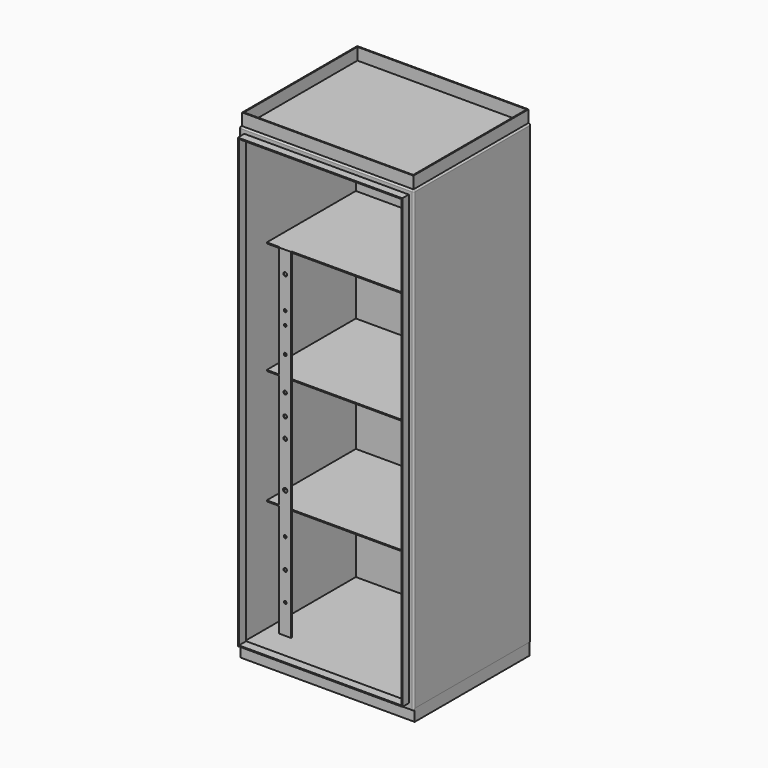
from build123d import *

# Parameters (mm, degrees)
F0_W          = 546.1
F0_H          = 1438.275
F1_DEPTH      = 3.175
F3_W          = 457.2
F3_H          = 1438.275
F4_DEPTH      = 3.175
F6_W          = 457.2
F6_H          = 1438.275
F7_DEPTH      = 3.175
F8_W          = 552.45
F8_H          = 457.2
F9_DEPTH      = 3.175
F10_W         = 546.1
F10_H         = 352.4375557899
F11_DEPTH     = 1.5875
F12_W         = 546.1
F12_H         = 352.425
F13_DEPTH     = 1.5875
F15_W         = 546.1
F15_H         = 352.425
F16_DEPTH     = 1.5875
F17_W         = 552.45
F17_H         = 457.2
F18_DEPTH     = 3.175
F20_DEPTH     = 2.54
F21_W         = 552.45
F21_H         = 1449.705
F21_W_2       = 514.35
F21_H_2       = 1411.605
F22_DEPTH     = 3.175
F23_W         = 520.7
F23_H         = 1417.955
F23_W_2       = 514.35
F23_H_2       = 1411.605
F24_DEPTH     = 25.4
F25_R         = 5.08
F26_T1_DEPTH  = 467.995
F26_S5_W      = 5.08
F26_S5_H      = 5.08
F26_T6_DEPTH  = 5.08
F26_S11_W     = 5.08
F26_S11_H     = 5.08
F26_T12_DEPTH = 5.08
F27_W         = 551.4826476574
F27_H         = 455.4039281793
F27_W_2       = 545.4865694046
F27_H_2       = 449.852083344
F28_DEPTH     = 38.1
F29_DEPTH     = 38.1
F30_W         = 542.29
F30_H         = 455.295
F30_W_2       = 535.94
F30_H_2       = 448.945
F31_DEPTH     = 38.1


# Not quite as in the source:
# - a fillet or chamfer that OpenCascade refuses, or shapes differently, is made with other operations: its cross-section is extruded or revolved along the edge and cut away or added


with BuildPart() as f1:
    # F0 (on Front) → F1 (new body)
    with BuildSketch(Plane.XZ):
        Rectangle(F0_W, F0_H)
    extrude(amount=-F1_DEPTH)

    # F3 (on face) → F4 (join)
    with BuildSketch(Plane.YZ.offset(273.05)):
        with Locations((-225.425, 0)):
            Rectangle(F3_W, F3_H)
    extrude(amount=F4_DEPTH)

    # F6 (on face) → F7 (join)
    with BuildSketch(Plane(origin=(-273.05, 0, 0), x_dir=(0, -1, 0), z_dir=(-1, 0, 0))):
        with Locations((225.425, 0)):
            Rectangle(F6_W, F6_H)
    extrude(amount=F7_DEPTH)

    # F8 (on face) → F9 (join)
    with BuildSketch(Plane(origin=(0, 0, -719.1375), x_dir=(1, 0, 0), z_dir=(0, 0, -1))):
        with Locations((0, 225.425)):
            Rectangle(F8_W, F8_H)
    extrude(amount=F9_DEPTH)

    # F10 (on offset) → F11 (join, symmetric)
    with BuildSketch(Plane.XY.offset(-363.5375)):
        with Locations((0, -176.218777895)):
            Rectangle(F10_W, F10_H)
    extrude(amount=F11_DEPTH, both=True)

    # F12 (on Top) → F13 (join, symmetric)
    with BuildSketch(Plane.XY):
        with Locations((0, -176.2125)):
            Rectangle(F12_W, F12_H)
    extrude(amount=F13_DEPTH, both=True)

    # F15 (on offset) → F16 (join, symmetric)
    with BuildSketch(Plane.XY.offset(355.6)):
        with Locations((0, -176.2125)):
            Rectangle(F15_W, F15_H)
    extrude(amount=F16_DEPTH, both=True)

    # F17 (on face) → F18 (join)
    with BuildSketch(Plane.XY.offset(719.1375)):
        with Locations((0, -225.425)):
            Rectangle(F17_W, F17_H)
    extrude(amount=F18_DEPTH)

    # F19 (on face) → F20 (join)
    with BuildSketch(Plane.XZ.offset(352.425)):
        with BuildLine():
            Line((-212.725, 357.1875), (-231.775, 357.1875))
            Line((-231.775, 357.1875), (-231.775, -719.3357628388))
            Line((-231.775, -719.3357628388), (-212.725, -719.3357628388))
            Line((-212.725, -719.3357628388), (-212.725, -630.4557702019))
            ThreePointArc((-212.725, -630.4557702019), (-217.117602153, -626.0631680489), (-212.725, -621.6705658958))
            Line((-212.725, -621.6705658958), (-212.725, -540.6397135398))
            ThreePointArc((-212.725, -540.6397135398), (-218.1377724311, -535.2269411087), (-212.725, -529.8141686776))
            Line((-212.725, -529.8141686776), (-212.725, -447.3259880815))
            ThreePointArc((-212.725, -447.3259880815), (-217.2657846247, -442.7852034569), (-212.725, -438.2444188322))
            Line((-212.725, -438.2444188322), (-212.725, -320.1060615697))
            ThreePointArc((-212.725, -320.1060615697), (-219.4191999116, -313.4118616581), (-212.725, -306.7176617465))
            Line((-212.725, -306.7176617465), (-212.725, -175.5880119798))
            ThreePointArc((-212.725, -175.5880119798), (-218.4829877374, -169.8300242424), (-212.725, -164.072036505))
            Line((-212.725, -164.072036505), (-212.725, -113.2661164384))
            ThreePointArc((-212.725, -113.2661164384), (-218.4185534458, -107.5725629926), (-212.725, -101.8790095467))
            Line((-212.725, -101.8790095467), (-212.725, -46.6509112122))
            ThreePointArc((-212.725, -46.6509112122), (-218.1210778716, -41.2548333406), (-212.725, -35.8587554691))
            Line((-212.725, -35.8587554691), (-212.725, 60.6955810605))
            ThreePointArc((-212.725, 60.6955810605), (-217.3495903553, 65.3201714158), (-212.725, 69.9447617711))
            Line((-212.725, 69.9447617711), (-212.725, 142.4734210846))
            ThreePointArc((-212.725, 142.4734210846), (-216.7484708908, 146.4968919754), (-212.725, 150.5203628662))
            Line((-212.725, 150.5203628662), (-212.725, 183.0033609852))
            ThreePointArc((-212.725, 183.0033609852), (-217.0262847916, 187.3046457767), (-212.725, 191.6059305683))
            Line((-212.725, 191.6059305683), (-212.725, 283.1353669526))
            ThreePointArc((-212.725, 283.1353669526), (-218.6943033336, 289.1046702862), (-212.725, 295.0739736198))
            Line((-212.725, 295.0739736198), (-212.725, 357.1875))
        make_face()
        with BuildLine():
            Line((-193.675, 357.1875), (-212.725, 357.1875))
            Line((-212.725, 357.1875), (-212.725, 295.0739736198))
            ThreePointArc((-212.725, 295.0739736198), (-208.5040651339, 293.3256051523), (-206.7556966664, 289.1046702862))
            ThreePointArc((-206.7556966664, 289.1046702862), (-208.5040651339, 284.88373542), (-212.725, 283.1353669526))
            Line((-212.725, 283.1353669526), (-212.725, 191.6059305683))
            ThreePointArc((-212.725, 191.6059305683), (-209.6835323561, 190.3461134207), (-208.4237152084, 187.3046457767))
            ThreePointArc((-208.4237152084, 187.3046457767), (-209.6835323561, 184.2631781328), (-212.725, 183.0033609852))
            Line((-212.725, 183.0033609852), (-212.725, 150.5203628662))
            ThreePointArc((-212.725, 150.5203628662), (-209.8799764492, 149.3419155262), (-208.7015291092, 146.4968919754))
            ThreePointArc((-208.7015291092, 146.4968919754), (-209.8799764492, 143.6518684246), (-212.725, 142.4734210846))
            Line((-212.725, 142.4734210846), (-212.725, 69.9447617711))
            ThreePointArc((-212.725, 69.9447617711), (-209.4549207996, 68.5902506162), (-208.1004096447, 65.3201714158))
            ThreePointArc((-208.1004096447, 65.3201714158), (-209.4549207996, 62.0500922154), (-212.725, 60.6955810605))
            Line((-212.725, 60.6955810605), (-212.725, -35.8587554691))
            ThreePointArc((-212.725, -35.8587554691), (-208.9093967452, -37.4392300858), (-207.3289221284, -41.2548333406))
            ThreePointArc((-207.3289221284, -41.2548333406), (-208.9093967452, -45.0704365955), (-212.725, -46.6509112122))
            Line((-212.725, -46.6509112122), (-212.725, -101.8790095467))
            ThreePointArc((-212.725, -101.8790095467), (-208.6990497494, -103.546612742), (-207.0314465542, -107.5725629926))
            ThreePointArc((-207.0314465542, -107.5725629926), (-208.6990497494, -111.5985132432), (-212.725, -113.2661164384))
            Line((-212.725, -113.2661164384), (-212.725, -164.072036505))
            ThreePointArc((-212.725, -164.072036505), (-208.6534878249, -165.7585120673), (-206.9670122626, -169.8300242424))
            ThreePointArc((-206.9670122626, -169.8300242424), (-208.6534878249, -173.9015364175), (-212.725, -175.5880119798))
            Line((-212.725, -175.5880119798), (-212.725, -306.7176617465))
            ThreePointArc((-212.725, -306.7176617465), (-207.9914858479, -308.678347506), (-206.0308000884, -313.4118616581))
            ThreePointArc((-206.0308000884, -313.4118616581), (-207.9914858479, -318.1453758102), (-212.725, -320.1060615697))
            Line((-212.725, -320.1060615697), (-212.725, -438.2444188322))
            ThreePointArc((-212.725, -438.2444188322), (-209.5141804, -439.5743838569), (-208.1842153753, -442.7852034569))
            ThreePointArc((-208.1842153753, -442.7852034569), (-209.5141804, -445.9960230569), (-212.725, -447.3259880815))
            Line((-212.725, -447.3259880815), (-212.725, -529.8141686776))
            ThreePointArc((-212.725, -529.8141686776), (-208.8975919089, -531.3995330176), (-207.3122275689, -535.2269411087))
            ThreePointArc((-207.3122275689, -535.2269411087), (-208.8975919089, -539.0543491998), (-212.725, -540.6397135398))
            Line((-212.725, -540.6397135398), (-212.725, -621.6705658958))
            ThreePointArc((-212.725, -621.6705658958), (-209.6189612305, -622.9571292794), (-208.332397847, -626.0631680489))
            ThreePointArc((-208.332397847, -626.0631680489), (-209.6189612305, -629.1692068183), (-212.725, -630.4557702019))
            Line((-212.725, -630.4557702019), (-212.725, -719.3357628388))
            Line((-212.725, -719.3357628388), (-193.675, -719.3357628388))
            Line((-193.675, -719.3357628388), (-193.675, 357.1875))
        make_face()
        with BuildLine():
            Line((231.775, -719.3357628388), (231.775, 357.1875))
            Line((231.775, 357.1875), (212.725, 357.1875))
            Line((212.725, 357.1875), (212.725, 295.2589705741))
            ThreePointArc((212.725, 295.2589705741), (217.0767474671, 293.4564177533), (218.879300288, 289.1046702862))
            ThreePointArc((218.879300288, 289.1046702862), (217.0767474671, 284.7529228191), (212.725, 282.9503699982))
            Line((212.725, 282.9503699982), (212.725, 195.2587648768))
            ThreePointArc((212.725, 195.2587648768), (218.349411554, 192.9290573307), (220.6791191, 187.3046457767))
            ThreePointArc((220.6791191, 187.3046457767), (218.349411554, 181.6802342227), (212.725, 179.3505266767))
            Line((212.725, 179.3505266767), (212.725, 152.5461312326))
            ThreePointArc((212.725, 152.5461312326), (217.0024580998, 150.7743500752), (218.7742392572, 146.4968919754))
            ThreePointArc((218.7742392572, 146.4968919754), (217.0024580998, 142.2194338756), (212.725, 140.4476527182))
            Line((212.725, 140.4476527182), (212.725, 72.6305128958))
            ThreePointArc((212.725, 72.6305128958), (217.8941920333, 70.4893634491), (220.03534148, 65.3201714158))
            ThreePointArc((220.03534148, 65.3201714158), (217.8941920333, 60.1509793825), (212.725, 58.0098299358))
            Line((212.725, 58.0098299358), (212.725, -35.4249250966))
            ThreePointArc((212.725, -35.4249250966), (216.847367653, -37.1324656876), (218.554908244, -41.2548333406))
            ThreePointArc((218.554908244, -41.2548333406), (216.847367653, -45.3772009937), (212.725, -47.0847415846))
            Line((212.725, -47.0847415846), (212.725, -102.0553301101))
            ThreePointArc((212.725, -102.0553301101), (216.6262727846, -103.671290208), (218.2422328825, -107.5725629926))
            ThreePointArc((218.2422328825, -107.5725629926), (216.6262727846, -111.4738357772), (212.725, -113.089795875))
            Line((212.725, -113.089795875), (212.725, -162.3801945495))
            ThreePointArc((212.725, -162.3801945495), (217.9928250946, -164.5621991478), (220.1748296929, -169.8300242424))
            ThreePointArc((220.1748296929, -169.8300242424), (217.9928250946, -175.097849337), (212.725, -177.2798539353))
            Line((212.725, -177.2798539353), (212.725, -306.509428103))
            ThreePointArc((212.725, -306.509428103), (217.6057575735, -308.5311040846), (219.6274335551, -313.4118616581))
            ThreePointArc((219.6274335551, -313.4118616581), (217.6057575735, -318.2926192316), (212.725, -320.3142952132))
            Line((212.725, -320.3142952132), (212.725, -436.1559807838))
            ThreePointArc((212.725, -436.1559807838), (217.4125683061, -438.0976351507), (219.3542226731, -442.7852034569))
            ThreePointArc((219.3542226731, -442.7852034569), (217.4125683061, -447.472771763), (212.725, -449.41442613))
            Line((212.725, -449.41442613), (212.725, -528.9798604641))
            ThreePointArc((212.725, -528.9798604641), (217.1423530864, -530.8095880223), (218.9720806446, -535.2269411087))
            ThreePointArc((218.9720806446, -535.2269411087), (217.1423530864, -539.6442941951), (212.725, -541.4740217533))
            Line((212.725, -541.4740217533), (212.725, -619.9717660694))
            ThreePointArc((212.725, -619.9717660694), (217.0322716466, -621.7558964023), (218.8164019794, -626.0631680489))
            ThreePointArc((218.8164019794, -626.0631680489), (217.0322716466, -630.3704396954), (212.725, -632.1545700283))
            Line((212.725, -632.1545700283), (212.725, -719.3357628388))
            Line((212.725, -719.3357628388), (231.775, -719.3357628388))
        make_face()
        with BuildLine():
            Line((212.725, 295.2589705741), (212.725, 357.1875))
            Line((212.725, 357.1875), (193.675, 357.1875))
            Line((193.675, 357.1875), (193.675, -719.3357628388))
            Line((193.675, -719.3357628388), (212.725, -719.3357628388))
            Line((212.725, -719.3357628388), (212.725, -632.1545700283))
            ThreePointArc((212.725, -632.1545700283), (206.6335980206, -626.0631680489), (212.725, -619.9717660694))
            Line((212.725, -619.9717660694), (212.725, -541.4740217533))
            ThreePointArc((212.725, -541.4740217533), (206.4779193554, -535.2269411087), (212.725, -528.9798604641))
            Line((212.725, -528.9798604641), (212.725, -449.41442613))
            ThreePointArc((212.725, -449.41442613), (206.0957773269, -442.7852034569), (212.725, -436.1559807838))
            Line((212.725, -436.1559807838), (212.725, -320.3142952132))
            ThreePointArc((212.725, -320.3142952132), (205.8225664449, -313.4118616581), (212.725, -306.509428103))
            Line((212.725, -306.509428103), (212.725, -177.2798539353))
            ThreePointArc((212.725, -177.2798539353), (205.2751703071, -169.8300242424), (212.725, -162.3801945495))
            Line((212.725, -162.3801945495), (212.725, -113.089795875))
            ThreePointArc((212.725, -113.089795875), (207.2077671175, -107.5725629926), (212.725, -102.0553301101))
            Line((212.725, -102.0553301101), (212.725, -47.0847415846))
            ThreePointArc((212.725, -47.0847415846), (206.895091756, -41.2548333406), (212.725, -35.4249250966))
            Line((212.725, -35.4249250966), (212.725, 58.0098299358))
            ThreePointArc((212.725, 58.0098299358), (205.41465852, 65.3201714158), (212.725, 72.6305128958))
            Line((212.725, 72.6305128958), (212.725, 140.4476527182))
            ThreePointArc((212.725, 140.4476527182), (206.6757607428, 146.4968919754), (212.725, 152.5461312326))
            Line((212.725, 152.5461312326), (212.725, 179.3505266767))
            ThreePointArc((212.725, 179.3505266767), (204.7708809, 187.3046457767), (212.725, 195.2587648768))
            Line((212.725, 195.2587648768), (212.725, 282.9503699982))
            ThreePointArc((212.725, 282.9503699982), (206.570699712, 289.1046702862), (212.725, 295.2589705741))
        make_face()
    extrude(amount=F20_DEPTH)

    # F21 (on face) → F22 (join)
    with BuildSketch(Plane.XZ.offset(454.025)):
        with Locations((0, -2.54)):
            Rectangle(F21_W, F21_H)
        with Locations((0, -2.54)):
            Rectangle(F21_W_2, F21_H_2, mode=Mode.SUBTRACT)
    extrude(amount=F22_DEPTH)

    # F23 (on face) → F24 (join)
    with BuildSketch(Plane.XZ.offset(457.2)):
        with Locations((0, -2.54)):
            Rectangle(F23_W, F23_H)
        with Locations((0, -2.54)):
            Rectangle(F23_W_2, F23_H_2, mode=Mode.SUBTRACT)
    extrude(amount=F24_DEPTH)

    # F25
    f25_edges = [f1.edges().sort_by_distance(p)[0] for p in [
        (0, -457.2, 722.3125),
        (276.225, -457.2, -2.54),
        (-276.225, -457.2, -2.54),
    ]]
    fillet(f25_edges, radius=F25_R)

    # F26: fillet of radius 5.08 on 2 edges, made by hand

    # F26_s2 → F26_t1 (cut)
    with BuildSketch(Plane.XZ.offset(-15.875)):
        with BuildLine():
            ThreePointArc((276.225, 717.2325), (274.7371024484, 720.8246024484), (271.145, 722.3125))
            Line((271.145, 722.3125), (276.225, 722.3125))
            Line((276.225, 722.3125), (276.225, 717.2325))
        make_face()
        with BuildLine():
            ThreePointArc((-276.225, 717.2325), (-274.7371024484, 720.8246024484), (-271.145, 722.3125))
            Line((-271.145, 722.3125), (-276.225, 722.3125))
            Line((-276.225, 722.3125), (-276.225, 717.2325))
        make_face()
    extrude(amount=F26_T1_DEPTH, mode=Mode.SUBTRACT)


with BuildPart() as f26_tool4:
    # F26_s5 → F26_t6 (new body)
    with BuildSketch(Plane.YZ.offset(-271.145)):
        with Locations((-454.66, 719.7725)):
            Rectangle(F26_S5_W, F26_S5_H)
    extrude(amount=-F26_T6_DEPTH)

    # F26_s7 → F26_t8 (revolve, cut)
    with BuildSketch(Plane(origin=(-271.145, -452.12, 717.2325), x_dir=(0, 0.7071067812, -0.7071067812), z_dir=(0, 0.7071067812, 0.7071067812))):
        with BuildLine():
            ThreePointArc((0, -5.08), (5.08, 0), (0, 5.08))
            Line((0, 5.08), (0, -5.08))
        make_face()
    revolve(axis=Axis((-271.145, -452.12, 717.2325), (-1, 0, 0)), mode=Mode.SUBTRACT)


with BuildPart() as f1_1:
    add(f1.part)

    # F26_t3: cut F26_tool4
    add(f26_tool4.part, mode=Mode.SUBTRACT)


with BuildPart() as f26_tool10:
    # F26_s11 → F26_t12 (new body)
    with BuildSketch(Plane.YZ.offset(271.145)):
        with Locations((-454.66, 719.7725)):
            Rectangle(F26_S11_W, F26_S11_H)
    extrude(amount=F26_T12_DEPTH)

    # F26_s13 → F26_t14 (revolve, cut)
    with BuildSketch(Plane(origin=(271.145, -452.12, 717.2325), x_dir=(0, 0.7071067812, -0.7071067812), z_dir=(0, -0.7071067812, -0.7071067812))):
        with BuildLine():
            ThreePointArc((0, -5.08), (5.08, 0), (0, 5.08))
            Line((0, 5.08), (0, -5.08))
        make_face()
    revolve(axis=Axis((271.145, -452.12, 717.2325), (1, 0, 0)), mode=Mode.SUBTRACT)


with BuildPart() as f1_2:
    add(f1_1.part)

    # F26_t9: cut F26_tool10
    add(f26_tool10.part, mode=Mode.SUBTRACT)

    # F27 (on face) → F28 (join)
    with BuildSketch(Plane(origin=(0, 0, -722.3125), x_dir=(1, 0, 0), z_dir=(0, 0, -1))):
        with Locations((0.0783056021, 225.4235425498)):
            Rectangle(F27_W, F27_H)
        with Locations((0.8957386017, 225.7214614656)):
            Rectangle(F27_W_2, F27_H_2, mode=Mode.SUBTRACT)
    extrude(amount=F28_DEPTH)

    # F27 (on face) → F29 (join)
    with BuildSketch(Plane(origin=(0, 0, -722.3125), x_dir=(1, 0, 0), z_dir=(0, 0, -1))):
        with Locations((0.0783056021, 225.4235425498)):
            Rectangle(F27_W, F27_H)
        with Locations((0.8957386017, 225.7214614656)):
            Rectangle(F27_W_2, F27_H_2, mode=Mode.SUBTRACT)
    extrude(amount=F29_DEPTH)

    # F30 (on face) → F31 (join)
    with BuildSketch(Plane.XY.offset(722.3125)):
        with Locations((0, -224.4725)):
            Rectangle(F30_W, F30_H)
        with Locations((0, -224.4725)):
            Rectangle(F30_W_2, F30_H_2, mode=Mode.SUBTRACT)
    extrude(amount=F31_DEPTH)


solid = f1_2.part
